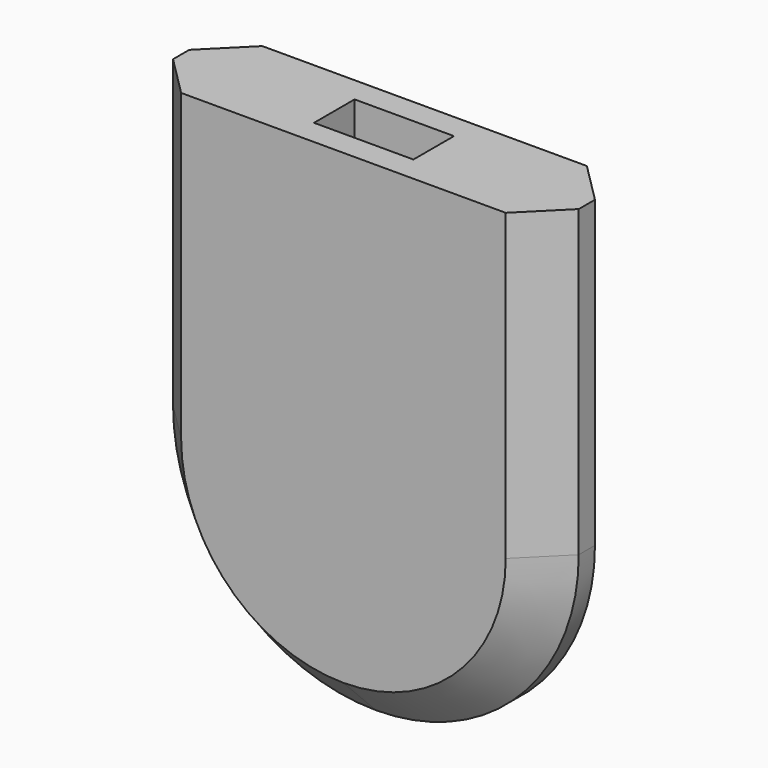
from build123d import *

# Parameters (mm, degrees)
F0_W     = 50.8
F0_H     = 12.7
F1_DEPTH = 25.4
F2_DEPTH = 63.5
F3_R     = 25.39999
F4_SIZE  = 5.08
F5_W     = 12.446
F5_H     = 6.35
F6_DEPTH = 25.4


# Not quite as in the source:
# - a fillet or chamfer is up to 0.001 mm smaller than in the source, because OpenCascade refuses the exact size


with BuildPart() as f1:
    # F0 (on Top) → F1 (new body)
    with BuildSketch(Plane.XY):
        Rectangle(F0_W, F0_H)
    extrude(amount=F1_DEPTH)

    # F0 (on Top) → F2 (join)
    with BuildSketch(Plane.XY):
        Rectangle(F0_W, F0_H)
    extrude(amount=F2_DEPTH)

    # F3 (radius 25.4 in the source; OpenCascade refuses exactly that, so slightly less here)
    f3_edges = [f1.edges().sort_by_distance(p)[0] for p in [
        (25.4, 0, 0),
        (-25.4, 0, 0),
    ]]
    fillet(f3_edges, radius=F3_R)

    # F4
    f4_edges = [f1.edges().sort_by_distance(p)[0] for p in [
        (-17.960515, -6.35, 7.439485),
        (-17.960515, 6.35, 7.439485),
    ]]
    chamfer(f4_edges, length=F4_SIZE)

    # F5 (on face) → F6 (cut)
    with BuildSketch(Plane.XY.offset(63.5)):
        Rectangle(F5_W, F5_H)
    extrude(amount=-F6_DEPTH, mode=Mode.SUBTRACT)


solid = f1.part
